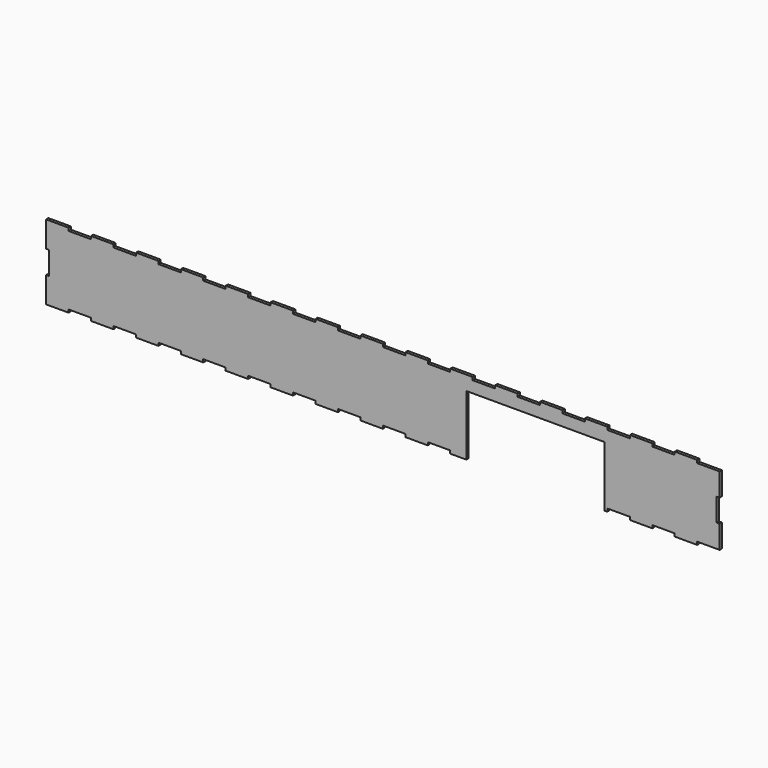
from build123d import *

# Parameters (mm, degrees)
F1_DEPTH = 3.175


# Not quite as in the source:
# - ends of sketch curves that miss each other by under 0.0002 mm in the source are joined


with BuildPart() as f1:
    # F0 (on Front) → F1 (new body)
    with BuildSketch(Plane.XZ):
        Polygon((92.075, 25.4), (244.475, 25.4), (244.475, -38.1), (244.475, -41.2750032454), (247.649968335, -41.2750032454), (247.649968335, -38.1000032454), (272.414968335, -38.1000032454), (272.414968335, -41.2750032454), (297.179968335, -41.2750032454), (297.179968335, -38.1000032454), (321.944968335, -38.1000032454), (321.944968335, -41.2750032454), (346.709968335, -41.2750032453), (346.709968335, -38.1000032454), (371.474968335, -38.0999963909), (371.475, -12.7), (368.3, -12.7), (368.3, 12.7), (371.475, 12.7), (371.475, 38.1), (368.3, 38.1), (346.7100335276, 38.1), (346.7100335276, 41.2750068545), (321.9450335276, 41.2750068544), (321.9450335276, 38.1000068545), (297.1800335276, 38.1000068545), (297.1800335276, 41.2750068545), (272.4150335276, 41.2750068545), (272.4150335276, 38.1000068545), (247.6500335276, 38.1000068545), (247.6500335276, 41.2750068545), (222.8850335276, 41.2750068545), (222.8850335276, 38.1000068545), (198.1200335276, 38.1000068545), (198.1200335276, 41.2750068545), (173.3550335276, 41.2750068545), (173.3550335276, 38.1000068545), (148.5900335276, 38.1000068545), (148.5900335276, 41.2750068545), (123.8250335276, 41.2750068545), (123.8250335276, 38.1000068545), (99.0600335276, 38.1000068545), (99.0600335276, 41.2750068545), (74.2950335276, 41.2750068545), (74.2950335276, 38.1000068545), (49.5300335276, 38.1000068545), (49.5300335276, 41.2750068545), (24.7650335276, 41.2750068545), (24.7650335276, 38.1000068545), (3.35276e-05, 38.1000068545), (3.35276e-05, 41.2750068545), (-24.7649664724, 41.2750068545), (-24.7649664724, 38.1000068545), (-49.5299664724, 38.1000068545), (-49.5299664724, 41.2750068545), (-74.2949664724, 41.2750068545), (-74.2949664724, 38.1000068545), (-99.0599664724, 38.1000068545), (-99.0599664724, 41.2750068545), (-123.8249664724, 41.2750068545), (-123.8249664724, 38.1000068545), (-148.5899664724, 38.1000068545), (-148.5899664724, 41.2750068545), (-173.3549664724, 41.2750068545), (-173.3549664724, 38.1000068545), (-198.1199664724, 38.1000068545), (-198.1199664724, 41.2750068545), (-222.8849664724, 41.2750068545), (-222.8849664724, 38.1000068545), (-247.6499664724, 38.1000068545), (-247.6499664724, 41.2750068545), (-272.4149664724, 41.2750068545), (-272.4149664724, 38.1000068545), (-297.1799664724, 38.1000068545), (-297.1799664724, 41.2750068545), (-321.9449664724, 41.2750068545), (-321.9449664724, 38.1000068545), (-346.7099664724, 38.1000068545), (-346.7099664724, 41.2750068545), (-371.4749664724, 41.2750068545), (-371.475, 38.1), (-371.475, 12.7), (-368.3, 12.7), (-368.3, -12.7), (-371.475, -12.7), (-371.475, -38.1), (-371.475031665, -41.2750032454), (-346.710031665, -41.2750032454), (-346.710031665, -38.1000032454), (-321.945031665, -38.1000032454), (-321.945031665, -41.2750032454), (-297.180031665, -41.2750032454), (-297.180031665, -38.1000032454), (-272.415031665, -38.1000032454), (-272.415031665, -41.2750032454), (-247.650031665, -41.2750032454), (-247.650031665, -38.1000032454), (-222.885031665, -38.1000032454), (-222.885031665, -41.2750032454), (-198.120031665, -41.2750032454), (-198.120031665, -38.1000032454), (-173.355031665, -38.1000032454), (-173.355031665, -41.2750032454), (-148.590031665, -41.2750032454), (-148.590031665, -38.1000032454), (-123.825031665, -38.1000032454), (-123.825031665, -41.2750032454), (-99.060031665, -41.2750032454), (-99.060031665, -38.1000032454), (-74.295031665, -38.1000032454), (-74.295031665, -41.2750032454), (-49.530031665, -41.2750032454), (-49.530031665, -38.1000032454), (-24.765031665, -38.1000032454), (-24.765031665, -41.2750032454), (-3.1665e-05, -41.2750032454), (-3.1665e-05, -38.1000032454), (24.764968335, -38.1000032454), (24.764968335, -41.2750032454), (49.529968335, -41.2750032454), (49.529968335, -38.1000032454), (74.294968335, -38.1000032454), (74.294968335, -41.2750032454), (92.075, -41.2750032454), (92.075, -38.1), align=None)
    extrude(amount=F1_DEPTH)


solid = f1.part
